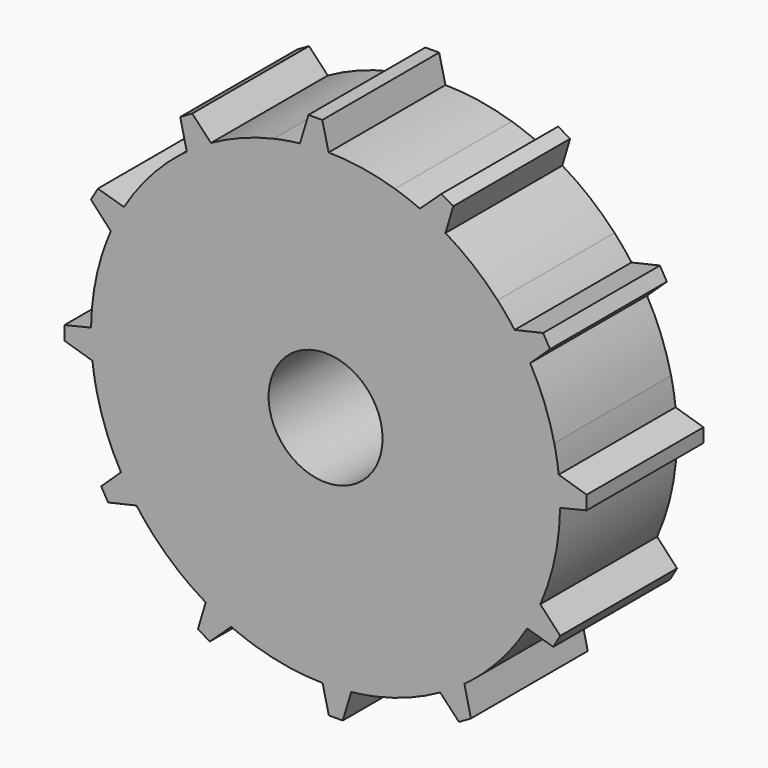
from build123d import *

# Parameters (mm, degrees)
F1_DEPTH = 25
F0_R     = 9.7528106777
F2_DEPTH = 25
F3_COUNT = 12


with BuildPart() as f1:
    # F0 (on Front) → F1 (new body)
    with BuildSketch(Plane.XZ):
        with BuildLine():
            ThreePointArc((35.2883561629, 1.0330273155), (27.4544642418, 24.8582881027), (7.0100539825, 39.385469638))
            ThreePointArc((7.0100539825, 39.385469638), (1.4007375004, 40.6889829464), (-4.3373688538, 41.1765419779))
            ThreePointArc((-4.3373688538, 41.1765419779), (-6.7990788962, 41.1329986982), (-9.2534905381, 40.9386386143))
            ThreePointArc((-9.2534905381, 40.9386386143), (-31.6478100439, -28.8686194646), (35.2883561629, 1.0330273155))
        make_face()
        with BuildLine():
            ThreePointArc((-4.85854148, 30.3700273155), (14.134700216, 22.5027690116), (22.00195852, 3.5095273155))
            ThreePointArc((22.00195852, 3.5095273155), (-22.4423355568, -16.7955618523), (-8.697145824, 30.0943270504))
            ThreePointArc((-8.697145824, 30.0943270504), (-6.7827876925, 30.3010135894), (-4.85854148, 30.3700273155))
        make_face(mode=Mode.SUBTRACT)
        with BuildLine():
            ThreePointArc((-9.2534905381, 40.9386386143), (-6.7990788962, 41.1329986982), (-4.3373688538, 41.1765419779))
            Line((-4.3373688538, 41.1765419779), (-5.4201926105, 45.7159504294))
            Line((-5.4201926105, 45.7159504294), (-7.7872149896, 45.7159504294))
            Line((-7.7872149896, 45.7159504294), (-9.2534905381, 40.9386386143))
        make_face()
    extrude(amount=F1_DEPTH)

    # F0 (on Front) → F2 (join)
    with BuildSketch(Plane.XZ):
        with BuildLine():
            ThreePointArc((-8.697145824, 30.0943270504), (-22.4423355568, -16.7955618523), (22.00195852, 3.5095273155))
            ThreePointArc((22.00195852, 3.5095273155), (14.134700216, 22.5027690116), (-4.85854148, 30.3700273155))
            ThreePointArc((-4.85854148, 30.3700273155), (-6.7827876925, 30.3010135894), (-8.697145824, 30.0943270504))
        make_face()
        with Locations((-4.85854148, 1.0330273155)):
            Circle(F0_R, mode=Mode.SUBTRACT)
    extrude(amount=F2_DEPTH)

    # F3: F1 ×12 about axis
    f3_axis = Axis((-4.85854148, 0, 1.0330273155), (0, -1, 0))


with BuildPart() as f1_1:
    add(f1.part)
    for i in range(1, F3_COUNT):
        add(f1.part.rotate(f3_axis, i * 360 / F3_COUNT))


solid = f1_1.part
